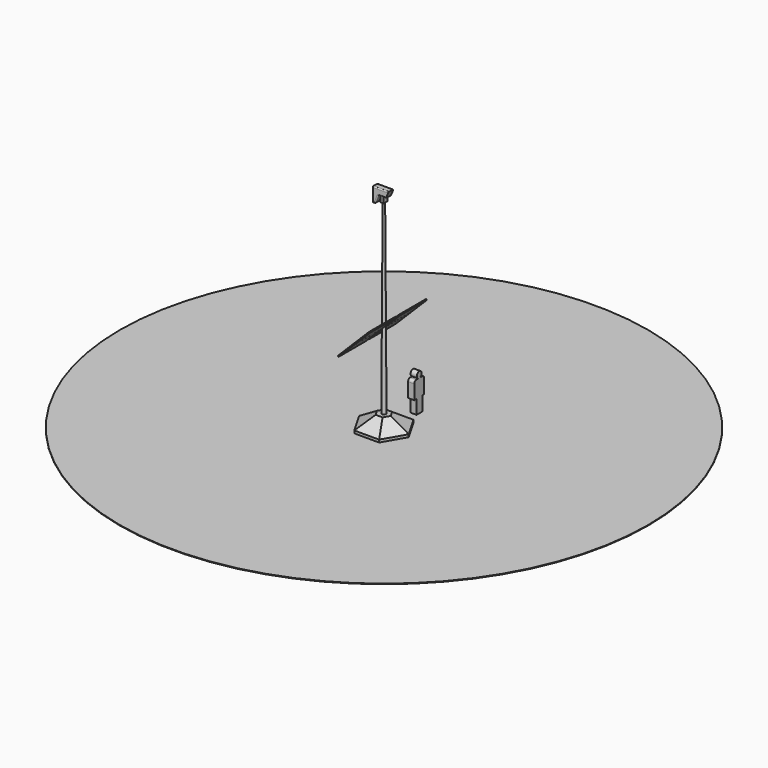
from build123d import *

# Parameters (mm, degrees)
F0_R          = 101.6
F2_R          = 48.26
F5_START      = 101.6
F5_DEPTH      = 1651
F6_T          = -4.1275
F11_DEPTH     = 635
F12_W         = 152.4
F12_H         = 254
F13_DEPTH     = 292.1
F15_DEPTH     = 152.4
F16_T1_DEPTH  = 304.8
F16_T3_DEPTH  = 1016
F16_T5_DEPTH  = 193.9775903579
F16_T7_DEPTH  = 367.3916007099
F16_T9_DEPTH  = 203.2
F16_T14_DEPTH = 51.816
F16_T20_DEPTH = 51.816
F16_T26_DEPTH = 473.3775903579
F16_T31_DEPTH = 473.3775903579
F16_T36_DEPTH = 473.3775903579
F16_T41_DEPTH = 473.3775903579
F16_T46_DEPTH = 473.3775903579
F16_T51_DEPTH = 473.3775903579
F16_T54_ANGLE = 68.5522636729
F16_T56_ANGLE = 68.5522636729
F17_SIZE2     = 508
F17_SIZE      = 762
F19_DEPTH     = 5.08
F20_R         = 12966.1709090086
F21_DEPTH     = 25.4
F23_DEPTH     = 304.8


# Not quite as in the source:
# - a fillet or chamfer that OpenCascade refuses, or shapes differently, is made with other operations: its cross-section is extruded or revolved along the edge and cut away or added


with BuildPart() as f3:
    # F0 (on Top) → F3 section 0
    with BuildSketch(Plane.XY):
        Circle(F0_R)
    # F2 (on offset) → F3 section 1
    with BuildSketch(Plane.XY.offset(9144)):
        Circle(F2_R)
    loft()

    # F6
    f6_openings = [f3.faces().sort_by_distance(p)[0] for p in [
        (0, 0, 9144),
        (0, 0, 0),
    ]]
    offset(amount=F6_T, openings=f6_openings, kind=Kind.INTERSECTION)

    # F12 (on face) → F13 (join)
    with BuildSketch(Plane.XY.offset(9144)):
        Rectangle(F12_W, F12_H)
    extrude(amount=F13_DEPTH)

    # F14 (on Front) → F15 (join, symmetric)
    with BuildSketch(Plane.XZ):
        Polygon((-76.2, 9436.1), (76.2, 9436.1), (228.6, 9436.1), (348.3428571429, 9740.9), (-413.6571428571, 9740.9), (-413.6571428571, 9029.7), (-312.0571428571, 9029.7), (-152.4, 9436.1), align=None)
    extrude(amount=F15_DEPTH, both=True)

    # F16: fillet of radius 50.8 on 10 edges, made by hand

    # F16_s2 → F16_t1 (join)
    with BuildSketch(Plane.XZ.offset(-152.4)):
        with BuildLine():
            ThreePointArc((-165.0597662246, 9403.8751405191), (-146.3872291325, 9427.2777151496), (-117.7775903579, 9436.1))
            Line((-117.7775903579, 9436.1), (-152.4, 9436.1))
            Line((-152.4, 9436.1), (-165.0597662246, 9403.8751405191))
        make_face()
    extrude(amount=F16_T1_DEPTH)

    # F16_s4 → F16_t3 (cut)
    with BuildSketch(Plane.YZ.offset(-540.6571428571)):
        with BuildLine():
            ThreePointArc((-152.4, 9690.1), (-137.5210244843, 9726.0210244843), (-101.6, 9740.9))
            Line((-101.6, 9740.9), (-152.4, 9740.9))
            Line((-152.4, 9740.9), (-152.4, 9690.1))
        make_face()
        with BuildLine():
            ThreePointArc((152.4, 9690.1), (137.5210244843, 9726.0210244843), (101.6, 9740.9))
            Line((101.6, 9740.9), (152.4, 9740.9))
            Line((152.4, 9740.9), (152.4, 9690.1))
        make_face()
    extrude(amount=F16_T3_DEPTH, mode=Mode.SUBTRACT)

    # F16_s6 → F16_t5 (cut)
    with BuildSketch(Plane.YZ.offset(-540.6571428571)):
        with BuildLine():
            ThreePointArc((-101.6, 9029.7), (-137.5210244843, 9044.5789755157), (-152.4, 9080.5))
            Line((-152.4, 9080.5), (-152.4, 9029.7))
            Line((-152.4, 9029.7), (-101.6, 9029.7))
        make_face()
        with BuildLine():
            ThreePointArc((101.6, 9029.7), (137.5210244843, 9044.5789755157), (152.4, 9080.5))
            Line((152.4, 9080.5), (152.4, 9029.7))
            Line((152.4, 9029.7), (101.6, 9029.7))
        make_face()
    extrude(amount=F16_T5_DEPTH, mode=Mode.SUBTRACT)

    # F16_s8 → F16_t7 (cut)
    with BuildSketch(Plane(origin=(3044.0284797211, 0, 7748.4361301991), x_dir=(0, 1, 0), z_dir=(0.3656523724, 0, 0.9307514934))):
        with BuildLine():
            ThreePointArc((-101.6, 3592.1788790209), (-137.5210244843, 3607.0578545367), (-152.4, 3642.9788790209))
            Line((-152.4, 3642.9788790209), (-152.4, 3592.1788790209))
            Line((-152.4, 3592.1788790209), (-101.6, 3592.1788790209))
        make_face()
        with BuildLine():
            ThreePointArc((101.6, 3592.1788790209), (137.5210244843, 3607.0578545367), (152.4, 3642.9788790209))
            Line((152.4, 3642.9788790209), (152.4, 3592.1788790209))
            Line((152.4, 3592.1788790209), (101.6, 3592.1788790209))
        make_face()
    extrude(amount=F16_T7_DEPTH, mode=Mode.SUBTRACT)

    # F16_s10 → F16_t9 (cut)
    with BuildSketch(Plane.XZ.offset(-101.6)):
        with BuildLine():
            ThreePointArc((-299.3973766325, 9061.9248594809), (-318.0699137246, 9038.5222848504), (-346.6795524993, 9029.7))
            Line((-346.6795524993, 9029.7), (-312.0571428571, 9029.7))
            Line((-312.0571428571, 9029.7), (-299.3973766325, 9061.9248594809))
        make_face()
    extrude(amount=F16_T9_DEPTH, mode=Mode.SUBTRACT)


with BuildPart() as f5:
    # F4 (on Front) → F5 (new body)
    with BuildSketch(Plane.XZ.offset(F5_START)):
        Polygon((-50.8, 3657.6), (703.5415141698, 4411.9415141698), (667.6204896855, 4447.8625386541), (-86.7210244843, 3693.5210244843), align=None)
    extrude(amount=F5_DEPTH)


with BuildPart() as f7_1:
    # F7: instance of F5
    add(f5.part.mirror(Plane.XZ))


with BuildPart() as f9_1:
    # F9: instance of F5
    add(f5.part.mirror(Plane(origin=(-77.7407683632, -927.1, 3666.5802561211), x_dir=(0, -1, 0), z_dir=(-0.7071067812, 0, -0.7071067812))))


with BuildPart() as f9_2:
    # F9: instance of F7_1
    add(f7_1.part.mirror(Plane(origin=(-77.7407683632, -927.1, 3666.5802561211), x_dir=(0, -1, 0), z_dir=(-0.7071067812, 0, -0.7071067812))))


with BuildPart() as f11:
    # F10 (on face) → F11 (new body)
    with BuildSketch(Plane(origin=(0, 0, 0), x_dir=(1, 0, 0), z_dir=(0, 0, -1))):
        Polygon((609.6, -1055.858172294), (1219.2, 0), (609.6, 1055.858172294), (-609.6, 1055.858172294), (-1219.2, 0), (-609.6, -1055.858172294), align=None)
    extrude(amount=F11_DEPTH)

    # F17
    f17_edges = [f11.edges().sort_by_distance(p)[0] for p in [
        (-914.4, 527.929086, 0),
        (-914.4, -527.929086, 0),
        (0, -1055.858172, 0),
        (914.4, -527.929086, 0),
        (914.4, 527.929086, 0),
        (0, 1055.858172, 0),
    ]]
    f17_side = f11.faces().sort_by_distance((0, 0, 0))[0]
    chamfer(f17_edges, length=F17_SIZE, length2=F17_SIZE2, reference=f17_side)


with BuildPart() as f16_tool12:
    # F16_s13 → F16_t14 (new body)
    with BuildSketch(Plane.XZ.offset(101.6)):
        Polygon((-346.6795524993, 9080.5), (-298.4517331152, 9061.5533566705), (-311.3646946643, 9028.684), (-346.6795524993, 9028.684), align=None)
    extrude(amount=F16_T14_DEPTH)

    # F16_s15 → F16_t16 (revolve, cut)
    with BuildSketch(Plane(origin=(-346.6795524993, -101.6, 9080.5), x_dir=(-0.5631818656, 0, 0.8263329754), z_dir=(0.8263329754, 0, 0.5631818656))):
        with BuildLine():
            ThreePointArc((0, -50.8), (50.8, 0), (0, 50.8))
            Line((0, 50.8), (0, -50.8))
        make_face()
    revolve(axis=Axis((-346.6795524993, -101.6, 9080.5), (0, -1, 0)), mode=Mode.SUBTRACT)


with BuildPart() as f3_1:
    add(f3.part)

    # F16_t11: cut F16_tool12
    add(f16_tool12.part, mode=Mode.SUBTRACT)


with BuildPart() as f16_tool18:
    # F16_s19 → F16_t20 (new body)
    with BuildSketch(Plane.XZ.offset(-101.6)):
        Polygon((-346.6795524993, 9080.5), (-298.4517331152, 9061.5533566705), (-311.3646946643, 9028.684), (-346.6795524993, 9028.684), align=None)
    extrude(amount=-F16_T20_DEPTH)

    # F16_s21 → F16_t22 (revolve, cut)
    with BuildSketch(Plane(origin=(-346.6795524993, 101.6, 9080.5), x_dir=(-0.5631818656, 0, 0.8263329754), z_dir=(-0.8263329754, 0, -0.5631818656))):
        with BuildLine():
            ThreePointArc((0, -50.8), (50.8, 0), (0, 50.8))
            Line((0, 50.8), (0, -50.8))
        make_face()
    revolve(axis=Axis((-346.6795524993, 101.6, 9080.5), (0, 1, 0)), mode=Mode.SUBTRACT)


with BuildPart() as f3_2:
    add(f3_1.part)

    # F16_t17: cut F16_tool18
    add(f16_tool18.part, mode=Mode.SUBTRACT)


with BuildPart() as f16_tool24:
    # F16_s25 → F16_t26 (new body)
    with BuildSketch(Plane.YZ.offset(355.6)):
        with BuildLine():
            ThreePointArc((-152.4, 9486.9), (-137.5210244843, 9450.9789755157), (-101.6, 9436.1))
            Line((-101.6, 9436.1), (-152.4, 9436.1))
            Line((-152.4, 9436.1), (-152.4, 9486.9))
        make_face()
    extrude(amount=-F16_T26_DEPTH)

    split(bisect_by=Plane.XZ.offset(127), keep=Keep.TOP)


with BuildPart() as f3_3:
    add(f3_2.part)

    # F16_t23: cut F16_tool24
    add(f16_tool24.part, mode=Mode.SUBTRACT)


with BuildPart() as f16_tool29:
    # F16_s30 → F16_t31 (new body)
    with BuildSketch(Plane.YZ.offset(355.6)):
        with BuildLine():
            ThreePointArc((-152.4, 9486.9), (-137.5210244843, 9450.9789755157), (-101.6, 9436.1))
            Line((-101.6, 9436.1), (-152.4, 9436.1))
            Line((-152.4, 9436.1), (-152.4, 9486.9))
        make_face()
    extrude(amount=-F16_T31_DEPTH)

    split(bisect_by=Plane.YZ.offset(76.2), keep=Keep.TOP)


with BuildPart() as f3_4:
    add(f3_3.part)

    # F16_t28: cut F16_tool29
    add(f16_tool29.part, mode=Mode.SUBTRACT)


with BuildPart() as f16_tool34:
    # F16_s35 → F16_t36 (new body)
    with BuildSketch(Plane.YZ.offset(355.6)):
        with BuildLine():
            ThreePointArc((-152.4, 9486.9), (-137.5210244843, 9450.9789755157), (-101.6, 9436.1))
            Line((-101.6, 9436.1), (-152.4, 9436.1))
            Line((-152.4, 9436.1), (-152.4, 9486.9))
        make_face()
    extrude(amount=-F16_T36_DEPTH)

    split(bisect_by=Plane.YZ.offset(-76.2), keep=Keep.BOTTOM)


with BuildPart() as f3_5:
    add(f3_4.part)

    # F16_t33: cut F16_tool34
    add(f16_tool34.part, mode=Mode.SUBTRACT)


with BuildPart() as f16_tool39:
    # F16_s40 → F16_t41 (new body)
    with BuildSketch(Plane.YZ.offset(-117.7775903579)):
        with BuildLine():
            ThreePointArc((152.4, 9486.9), (137.5210244843, 9450.9789755157), (101.6, 9436.1))
            Line((101.6, 9436.1), (152.4, 9436.1))
            Line((152.4, 9436.1), (152.4, 9486.9))
        make_face()
    extrude(amount=F16_T41_DEPTH)

    split(bisect_by=Plane.XZ.offset(-127), keep=Keep.BOTTOM)


with BuildPart() as f3_6:
    add(f3_5.part)

    # F16_t38: cut F16_tool39
    add(f16_tool39.part, mode=Mode.SUBTRACT)


with BuildPart() as f16_tool44:
    # F16_s45 → F16_t46 (new body)
    with BuildSketch(Plane.YZ.offset(-117.7775903579)):
        with BuildLine():
            ThreePointArc((152.4, 9486.9), (137.5210244843, 9450.9789755157), (101.6, 9436.1))
            Line((101.6, 9436.1), (152.4, 9436.1))
            Line((152.4, 9436.1), (152.4, 9486.9))
        make_face()
    extrude(amount=F16_T46_DEPTH)

    split(bisect_by=Plane.YZ.offset(-76.2), keep=Keep.BOTTOM)


with BuildPart() as f3_7:
    add(f3_6.part)

    # F16_t43: cut F16_tool44
    add(f16_tool44.part, mode=Mode.SUBTRACT)


with BuildPart() as f16_tool49:
    # F16_s50 → F16_t51 (new body)
    with BuildSketch(Plane.YZ.offset(-117.7775903579)):
        with BuildLine():
            ThreePointArc((152.4, 9486.9), (137.5210244843, 9450.9789755157), (101.6, 9436.1))
            Line((101.6, 9436.1), (152.4, 9436.1))
            Line((152.4, 9436.1), (152.4, 9486.9))
        make_face()
    extrude(amount=F16_T51_DEPTH)

    split(bisect_by=Plane.YZ.offset(76.2), keep=Keep.TOP)


with BuildPart() as f3_8:
    add(f3_7.part)

    # F16_t48: cut F16_tool49
    add(f16_tool49.part, mode=Mode.SUBTRACT)

    # F16_s53 → F16_t54 (revolve, cut)
    with BuildSketch(Plane(origin=(3178.3660901289, 0, 8090.3864112374), x_dir=(0, 1, 0), z_dir=(-0.3656523724, 0, -0.9307514934))):
        with BuildLine():
            ThreePointArc((101.6, -3592.1788790208), (137.5210244843, -3607.0578545366), (152.4, -3642.9788790208))
            Line((152.4, -3642.9788790208), (152.4, -3592.1788790208))
            Line((152.4, -3592.1788790208), (101.6, -3592.1788790208))
        make_face()
    revolve(axis=Axis((-117.7775903579, 152.4, 9385.3), (0, 1, 0)), revolution_arc=F16_T54_ANGLE, mode=Mode.SUBTRACT)

    # F16_s55 → F16_t56 (revolve, cut)
    with BuildSketch(Plane(origin=(3178.3660901289, 0, 8090.3864112374), x_dir=(0, 1, 0), z_dir=(-0.3656523724, 0, -0.9307514934))):
        with BuildLine():
            ThreePointArc((-152.4, -3642.9788790208), (-137.5210244843, -3607.0578545366), (-101.6, -3592.1788790208))
            Line((-101.6, -3592.1788790208), (-152.4, -3592.1788790208))
            Line((-152.4, -3592.1788790208), (-152.4, -3642.9788790208))
        make_face()
    revolve(axis=Axis((-117.7775903579, -152.4, 9385.3), (0, 1, 0)), revolution_arc=F16_T56_ANGLE, mode=Mode.SUBTRACT)


with BuildPart() as f19:
    # F18 (on face) → F19 (new body)
    with BuildSketch(Plane(origin=(-413.6571428571, 0, 0), x_dir=(0, -1, 0), z_dir=(-1, 0, 0))):
        with BuildLine():
            ThreePointArc((152.4, 9690.1), (137.5210244843, 9726.0210244843), (101.6, 9740.9))
            Line((101.6, 9740.9), (-101.6, 9740.9))
            ThreePointArc((-101.6, 9740.9), (-137.5210244843, 9726.0210244843), (-152.4, 9690.1))
            Line((-152.4, 9690.1), (-152.4, 9080.5))
            ThreePointArc((-152.4, 9080.5), (-137.5210244843, 9044.5789755157), (-101.6, 9029.7))
            Line((-101.6, 9029.7), (101.6, 9029.7))
            ThreePointArc((101.6, 9029.7), (137.5210244843, 9044.5789755157), (152.4, 9080.5))
            Line((152.4, 9080.5), (152.4, 9690.1))
        make_face()
    extrude(amount=F19_DEPTH)


with BuildPart() as f21:
    # F20 (on face) → F21 (new body)
    with BuildSketch(Plane(origin=(0, 0, -635), x_dir=(1, 0, 0), z_dir=(0, 0, -1))):
        with Locations((-26.8027372658, -39.2579697073)):
            Circle(F20_R)
    extrude(amount=F21_DEPTH)


with BuildPart() as f23:
    # F22 (on Right) → F23 (new body)
    with BuildSketch(Plane.YZ):
        with BuildLine():
            Line((1965.0307300568, 897.2154969875), (1836.5925482063, 897.2154969875))
            ThreePointArc((1836.5925482063, 897.2154969875), (1787.2307300568, 1193.8), (1737.8689119073, 897.2154969875))
            Line((1737.8689119073, 897.2154969875), (1609.4307300568, 897.2154969875))
            ThreePointArc((1609.4307300568, 897.2154969875), (1519.6281688461, 860.0180581981), (1482.4307300568, 770.2154969875))
            Line((1482.4307300568, 770.2154969875), (1482.4307300568, 61.6458617151))
            Line((1482.4307300568, 61.6458617151), (1624.8757839203, 61.6458617151))
            Line((1624.8757839203, 61.6458617151), (1624.8757839203, -628.3607368764))
            Line((1624.8757839203, -628.3607368764), (1980.3770780563, -628.3607368764))
            Line((1980.3770780563, -628.3607368764), (1980.3770780563, 67.2442913055))
            Line((1980.3770780563, 67.2442913055), (2092.0307300568, 67.2442913055))
            Line((2092.0307300568, 67.2442913055), (2092.0307300568, 770.2154969875))
            ThreePointArc((2092.0307300568, 770.2154969875), (2054.8332912675, 860.0180581981), (1965.0307300568, 897.2154969875))
        make_face()
    extrude(amount=F23_DEPTH)


solid = Compound([f5.part, f7_1.part, f9_1.part, f9_2.part, f11.part, f3_8.part, f19.part, f21.part, f23.part])
